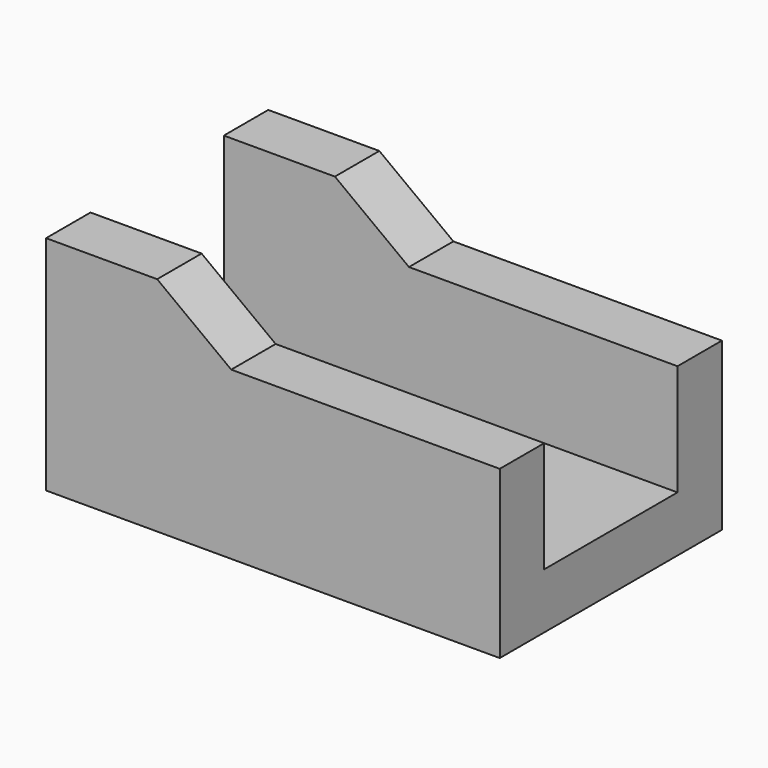
from build123d import *

# Parameters (mm, degrees)
F0_W     = 77.8002
F0_H     = 47.625
F1_DEPTH = 9.525
F3_DEPTH = 9.525


# Not quite as in the source:
# - a pattern or mirror of a feature is missing from the dataset's text; its kind, count and spacing are read off the source's solid


with BuildPart() as f1:
    # F0 (on Top) → F1 (new body)
    with BuildSketch(Plane.XY):
        Rectangle(F0_W, F0_H)
    extrude(amount=F1_DEPTH)

    # F2 (on face) → F3 (join)
    with BuildSketch(Plane.XZ.offset(23.8125)):
        Polygon((-38.9001, 38.1), (-38.9001, 9.525), (38.9001, 9.525), (38.9001, 28.575), (-7.1501, 28.575), (-19.8501, 38.1), align=None)
    f3 = extrude(amount=-F3_DEPTH)

    # F3_copies: F3 across plane
    add(f3.mirror(Plane.ZX))


solid = f1.part
